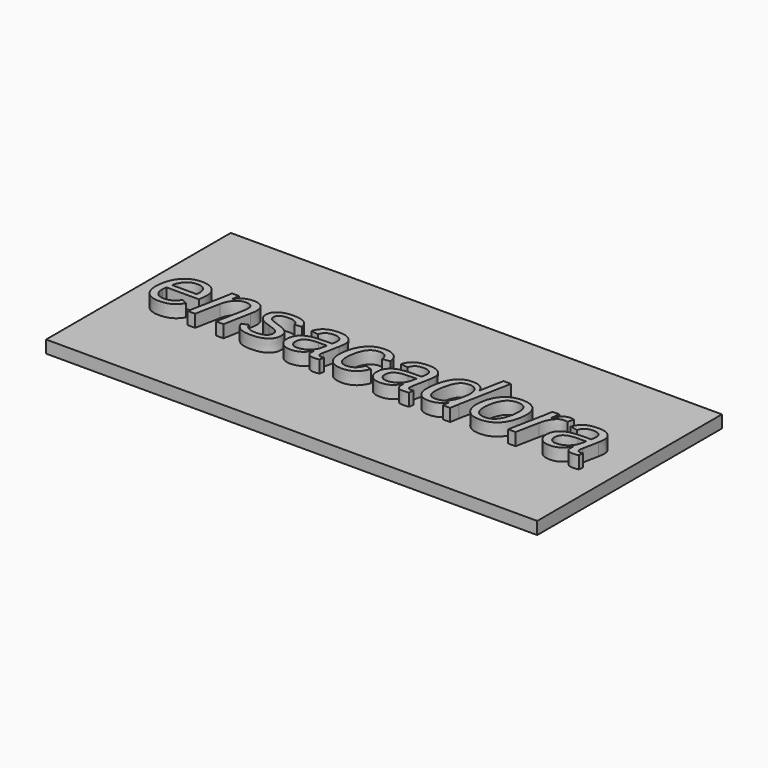
from build123d import *

# Parameters (mm, degrees)
F0_W         = 1000
F0_H         = 470
F1_DEPTH     = 25.4
F2_TEXT_SIZE = 172.5660950246
F3_DEPTH     = 25.4


# Not quite as in the source:
# - Text() gives the source's letters only with a copy of the font that has no kerning and outlines rounded to 1/6400 em; it was checked with that copy


with BuildPart() as f1:
    # F0 (on Top) → F1 (new body)
    with BuildSketch(Plane.XY):
        Rectangle(F0_W, F0_H)
    extrude(amount=F1_DEPTH)

    # F2 (on face) → F3 (join)
    with BuildSketch(Plane.XY.offset(25.4)):
        with Locations((-453.9297202718, -55.7292673484)):
            Text('ensacadora', F2_TEXT_SIZE, font='Arimo', font_style=FontStyle.ITALIC, text_align=(TextAlign.LEFT, TextAlign.BOTTOM))
    extrude(amount=F3_DEPTH)


solid = f1.part
